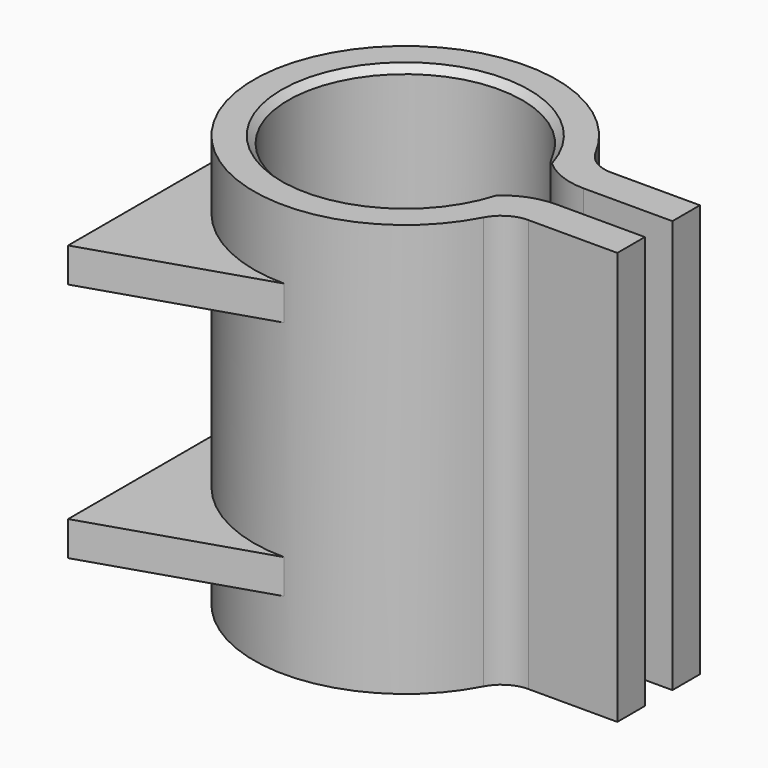
from build123d import *

# Parameters (mm, degrees)
F1_DEPTH    = 30
F2_T2_ANGLE = 334.4485965255
F2_T4_ANGLE = 334.4485965255
F4_START    = -10
F4_DEPTH    = 5


# Not quite as in the source:
# - a fillet or chamfer that OpenCascade refuses, or shapes differently, is made with other operations: its cross-section is extruded or revolved along the edge and cut away or added


with BuildPart() as f1:
    # F0 (on Top) → F1 (new body, symmetric)
    with BuildSketch(Plane.XY):
        with BuildLine():
            ThreePointArc((15.0684196329, -7.8703703704), (-17, 0), (15.0684196329, 7.8703703704))
            ThreePointArc((15.0684196329, 7.8703703704), (18.7503186358, 3.9473309343), (23.9321958875, 2.5))
            Line((23.9321958875, 2.5), (36.8151717208, 2.5))
            Line((36.8151717208, 2.5), (36.8151717208, 7.5))
            Line((36.8151717208, 7.5), (23.9321958875, 7.5))
            ThreePointArc((23.9321958875, 7.5), (21.3412572617, 8.2236654671), (19.5003077602, 10.1851851852))
            ThreePointArc((19.5003077602, 10.1851851852), (-22, 0), (19.5003077602, -10.1851851852))
            ThreePointArc((19.5003077602, -10.1851851852), (21.3412572617, -8.2236654671), (23.9321958875, -7.5))
            Line((23.9321958875, -7.5), (36.8151717208, -7.5))
            Line((36.8151717208, -7.5), (36.8151717208, -2.5))
            Line((36.8151717208, -2.5), (23.9321958875, -2.5))
            ThreePointArc((23.9321958875, -2.5), (18.7503186358, -3.9473309343), (15.0684196329, -7.8703703704))
        make_face()
    extrude(amount=F1_DEPTH, both=True)

    # F2: chamfer of 1 on 2 edges, made by hand

    # F2_s1 → F2_t2 (revolve, cut)
    with BuildSketch(Plane(origin=(0, 0, 0), x_dir=(0, 0, 1), z_dir=(0.2211349318, 0.9752432219, 0))):
        Polygon((30, 18), (29, 17), (30, 17), align=None)
    revolve(axis=Axis((0, 0, 30), (0, 0, -1)), revolution_arc=F2_T2_ANGLE, mode=Mode.SUBTRACT)

    # F2_s3 → F2_t4 (revolve, cut)
    with BuildSketch(Plane(origin=(0, 0, 0), x_dir=(0, 0, 1), z_dir=(0.2211349318, 0.9752432219, 0))):
        Polygon((-29, 17), (-30, 18), (-30, 17), align=None)
    revolve(axis=Axis((0, 0, -30), (0, 0, -1)), revolution_arc=F2_T4_ANGLE, mode=Mode.SUBTRACT)

    # F3 (on face) → F4 (join)
    with BuildSketch(Plane(origin=(0, 0, -30), x_dir=(1, 0, 0), z_dir=(0, 0, -1)).offset(F4_START)):
        with BuildLine():
            ThreePointArc((0, -22), (-22, 0), (0, 22))
            Line((0, 22), (-25, 30))
            Line((-25, 30), (-25, -30))
            Line((-25, -30), (0, -22))
        make_face()
    extrude(amount=-F4_DEPTH)

    # F5: F1 across plane


with BuildPart() as f1_1:
    add(f1.part)
    add(f1.part.mirror(Plane.XY))


solid = f1_1.part
